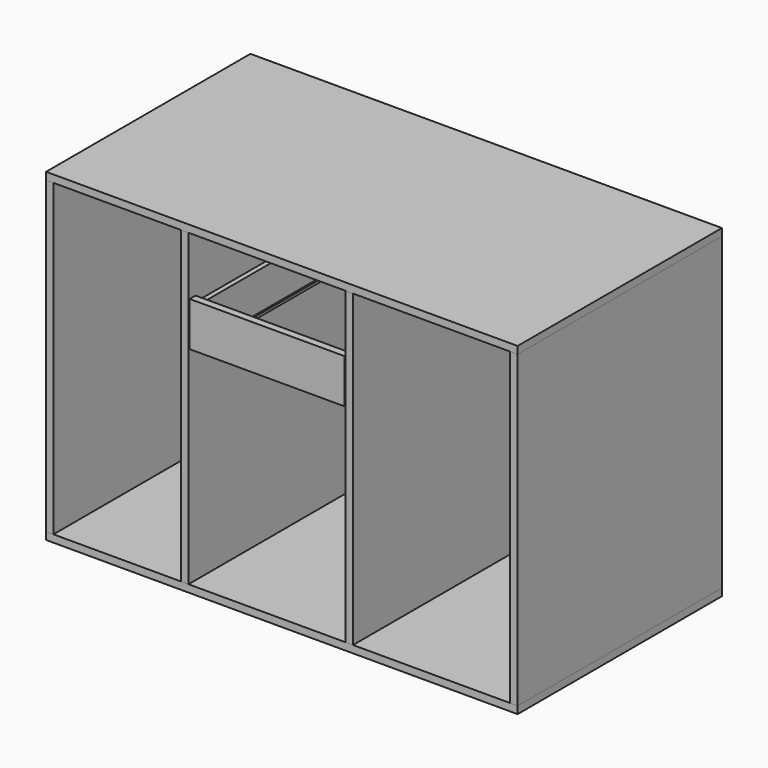
from build123d import *

# Parameters (mm, degrees)
F0_W     = 1219.2
F0_H     = 660.4
F1_DEPTH = 19.05
F2_W     = 19.05
F2_H     = 660.4
F3_DEPTH = 800.1
F4_W     = 1219.2
F4_H     = 660.4
F5_DEPTH = 19.05
F6_W     = 400.05
F6_H     = 114.3
F7_DEPTH = 19.05
F9_DEPTH = 635


# Not quite as in the source:
# - a length typed as a fraction of an inch, garbled in the dataset ("3 / 203.2 mm" for 3/8 in), is restored


with BuildPart() as f1:
    # F0 (on Top) → F1 (new body)
    with BuildSketch(Plane.XY):
        with Locations((5.564596504, 40.9429918908)):
            Rectangle(F0_W, F0_H)
    extrude(amount=F1_DEPTH)


with BuildPart() as f3:
    # F2 (on face) → F3 (new body)
    with BuildSketch(Plane(origin=(0, 0, 0), x_dir=(1, 0, 0), z_dir=(0, 0, -1))):
        with Locations((-594.510403496, -40.9429918908)):
            Rectangle(F2_W, F2_H)
    extrude(amount=F3_DEPTH)


with BuildPart() as f3b:
    # F2 (on face) → F3, piece 2 (new body)
    with BuildSketch(Plane(origin=(0, 0, 0), x_dir=(1, 0, 0), z_dir=(0, 0, -1))):
        with Locations((605.639596504, -40.9429918908)):
            Rectangle(F2_W, F2_H)
    extrude(amount=F3_DEPTH)


with BuildPart() as f3c:
    # F2 (on face) → F3, piece 3 (new body)
    with BuildSketch(Plane(origin=(0, 0, 0), x_dir=(1, 0, 0), z_dir=(0, 0, -1))):
        with Locations((180.189596504, -40.9429918908)):
            Rectangle(F2_W, F2_H)
    extrude(amount=F3_DEPTH)


with BuildPart() as f3d:
    # F2 (on face) → F3, piece 4 (new body)
    with BuildSketch(Plane(origin=(0, 0, 0), x_dir=(1, 0, 0), z_dir=(0, 0, -1))):
        with Locations((-245.260403496, -40.9429918908)):
            Rectangle(F2_W, F2_H)
    extrude(amount=F3_DEPTH)


with BuildPart() as f5:
    # F4 (on face) → F5 (new body)
    with BuildSketch(Plane(origin=(0, 0, -800.1), x_dir=(1, 0, 0), z_dir=(0, 0, -1))):
        with Locations((5.564596504, -40.9429918908)):
            Rectangle(F4_W, F4_H)
    extrude(amount=F5_DEPTH)


with BuildPart() as f7:
    # F6 (on face) → F7 (new body)
    with BuildSketch(Plane.XZ.offset(289.2570081092)):
        with Locations((-32.535403496, -206.838673687)):
            Rectangle(F6_W, F6_H)
    extrude(amount=-F7_DEPTH)


with BuildPart() as f9:
    # F8 (on face) → F9 (new body)
    with BuildSketch(Plane(origin=(0, -270.2070081092, 0), x_dir=(-1, 0, 0), z_dir=(0, 1, 0))):
        Polygon((-145.264596504, -156.038673687), (-157.964596504, -156.038673687), (-157.964596504, -263.988673687), (-145.264596504, -263.988673687), (-145.264596504, -257.638673687), (-151.614596504, -257.638673687), (-151.614596504, -253.669923687), (-145.264596504, -253.669923687), align=None)
    extrude(amount=F9_DEPTH)


with BuildPart() as f9b:
    # F8 (on face) → F9, piece 2 (new body)
    with BuildSketch(Plane(origin=(0, -270.2070081092, 0), x_dir=(-1, 0, 0), z_dir=(0, 1, 0))):
        Polygon((216.685403496, -253.669923687), (216.685403496, -257.638673687), (210.335403496, -257.638673687), (210.335403496, -263.988673687), (223.035403496, -263.988673687), (223.035403496, -156.038673687), (210.335403496, -156.038673687), (210.335403496, -253.669923687), align=None)
    extrude(amount=F9_DEPTH)


solid = Compound([f1.part, f3.part, f3b.part, f3c.part, f3d.part, f5.part, f7.part, f9.part, f9b.part])
